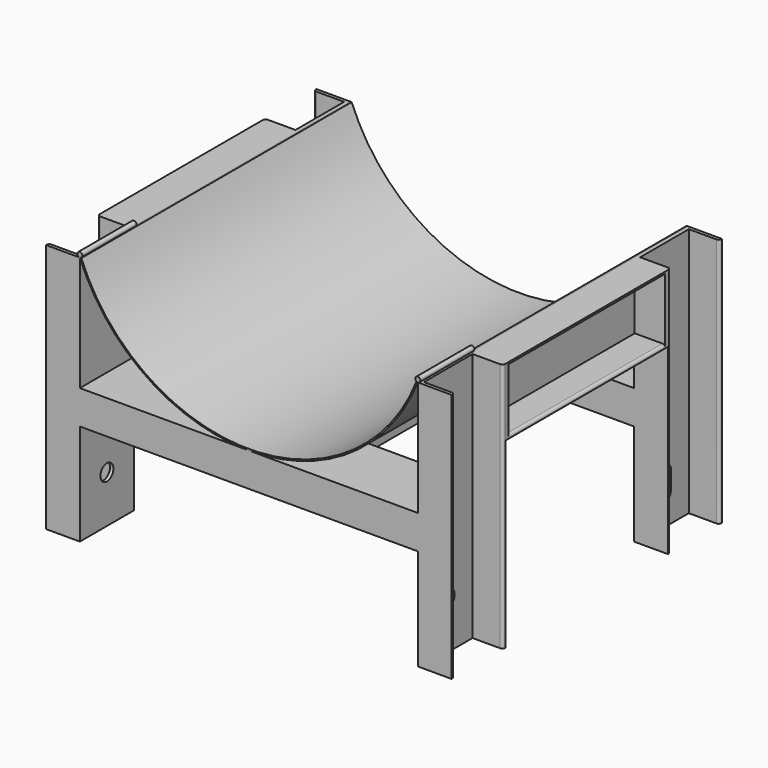
from build123d import *

# Parameters (mm, degrees)
F0_W      = 100
F0_H      = 150
F1_DEPTH  = 50
F2_T      = -5
F3_DEPTH  = 170
F4_DEPTH  = 200
F7_DEPTH  = 250
F8_W      = 300
F8_H      = 100
F9_DEPTH  = 50
F10_T     = -5
F11_R     = 4
F14_DEPTH = 555.001
F15_D     = 24
F16_R     = 3.75
F17_DEPTH = 100


# Not quite as in the source:
# - a feature names something its author has since deleted; it is built from what else it names


with BuildPart() as f1:
    # F0 (on Top) → F1 (new body)
    with BuildSketch(Plane.XY):
        Polygon((250, 250), (-250, 250), (-250, 150), (-50, 150), (50, 150), (250, 150), align=None)
        with Locations((0, 75)):
            Rectangle(F0_W, F0_H)
        with Locations((0, -75)):
            Rectangle(F0_W, F0_H)
        Polygon((50, -150), (-50, -150), (-250, -150), (-250, -250), (250, -250), (250, -150), align=None)
    extrude(amount=-F1_DEPTH)

    # F2
    f2_openings = [f1.faces().sort_by_distance(p)[0] for p in [
        (0, 0, -50),
    ]]
    offset(amount=F2_T, openings=f2_openings, kind=Kind.INTERSECTION)


with BuildPart() as f3:
    # F0 (on Top) → F3 (new body)
    with BuildSketch(Plane.XY):
        with BuildLine():
            Line((-250, -250), (-250, -150))
            Line((-250, -150), (-300, -150))
            Line((-300, -150), (-300, -151))
            ThreePointArc((-300, -151), (-298.8284271247, -153.8284271247), (-296, -155))
            Line((-296, -155), (-255, -155))
            Line((-255, -155), (-255, -245))
            Line((-255, -245), (-296, -245))
            ThreePointArc((-296, -245), (-298.8284271247, -246.1715728753), (-300, -249))
            Line((-300, -249), (-300, -250))
            Line((-300, -250), (-250, -250))
        make_face()
    extrude(amount=F3_DEPTH)


with BuildPart() as f3b:
    # F0 (on Top) → F3, piece 2 (new body)
    with BuildSketch(Plane.XY):
        with BuildLine():
            Line((300, -150), (250, -150))
            Line((250, -150), (250, -250))
            Line((250, -250), (300, -250))
            Line((300, -250), (300, -249))
            ThreePointArc((300, -249), (298.8284271247, -246.1715728753), (296, -245))
            Line((296, -245), (255, -245))
            Line((255, -245), (255, -155))
            Line((255, -155), (296, -155))
            ThreePointArc((296, -155), (298.8284271247, -153.8284271247), (300, -151))
            Line((300, -151), (300, -150))
        make_face()
    extrude(amount=F3_DEPTH)


with BuildPart() as f3c:
    # F0 (on Top) → F3, piece 3 (new body)
    with BuildSketch(Plane.XY):
        with BuildLine():
            Line((300, 250), (250, 250))
            Line((250, 250), (250, 150))
            Line((250, 150), (300, 150))
            Line((300, 150), (300, 151))
            ThreePointArc((300, 151), (298.8284271247, 153.8284271247), (296, 155))
            Line((296, 155), (255, 155))
            Line((255, 155), (255, 245))
            Line((255, 245), (296, 245))
            ThreePointArc((296, 245), (298.8284271247, 246.1715728753), (300, 249))
            Line((300, 249), (300, 250))
        make_face()
    extrude(amount=F3_DEPTH)


with BuildPart() as f3d:
    # F0 (on Top) → F3, piece 4 (new body)
    with BuildSketch(Plane.XY):
        with BuildLine():
            Line((-250, 150), (-250, 250))
            Line((-250, 250), (-300, 250))
            Line((-300, 250), (-300, 249))
            ThreePointArc((-300, 249), (-298.8284271247, 246.1715728753), (-296, 245))
            Line((-296, 245), (-255, 245))
            Line((-255, 245), (-255, 155))
            Line((-255, 155), (-296, 155))
            ThreePointArc((-296, 155), (-298.8284271247, 153.8284271247), (-300, 151))
            Line((-300, 151), (-300, 150))
            Line((-300, 150), (-250, 150))
        make_face()
    extrude(amount=F3_DEPTH)


with BuildPart() as f4:
    # F0 (on Top) → F4 (new body)
    with BuildSketch(Plane.XY):
        with BuildLine():
            Line((-250, -250), (-250, -150))
            Line((-250, -150), (-300, -150))
            Line((-300, -150), (-300, -151))
            ThreePointArc((-300, -151), (-298.8284271247, -153.8284271247), (-296, -155))
            Line((-296, -155), (-255, -155))
            Line((-255, -155), (-255, -245))
            Line((-255, -245), (-296, -245))
            ThreePointArc((-296, -245), (-298.8284271247, -246.1715728753), (-300, -249))
            Line((-300, -249), (-300, -250))
            Line((-300, -250), (-250, -250))
        make_face()
    extrude(amount=-F4_DEPTH)


with BuildPart() as f4b:
    # F0 (on Top) → F4, piece 2 (new body)
    with BuildSketch(Plane.XY):
        with BuildLine():
            Line((300, -150), (250, -150))
            Line((250, -150), (250, -250))
            Line((250, -250), (300, -250))
            Line((300, -250), (300, -249))
            ThreePointArc((300, -249), (298.8284271247, -246.1715728753), (296, -245))
            Line((296, -245), (255, -245))
            Line((255, -245), (255, -155))
            Line((255, -155), (296, -155))
            ThreePointArc((296, -155), (298.8284271247, -153.8284271247), (300, -151))
            Line((300, -151), (300, -150))
        make_face()
    extrude(amount=-F4_DEPTH)


with BuildPart() as f4c:
    # F0 (on Top) → F4, piece 3 (new body)
    with BuildSketch(Plane.XY):
        with BuildLine():
            Line((300, 250), (250, 250))
            Line((250, 250), (250, 150))
            Line((250, 150), (300, 150))
            Line((300, 150), (300, 151))
            ThreePointArc((300, 151), (298.8284271247, 153.8284271247), (296, 155))
            Line((296, 155), (255, 155))
            Line((255, 155), (255, 245))
            Line((255, 245), (296, 245))
            ThreePointArc((296, 245), (298.8284271247, 246.1715728753), (300, 249))
            Line((300, 249), (300, 250))
        make_face()
    extrude(amount=-F4_DEPTH)


with BuildPart() as f4d:
    # F0 (on Top) → F4, piece 4 (new body)
    with BuildSketch(Plane.XY):
        with BuildLine():
            Line((-250, 150), (-250, 250))
            Line((-250, 250), (-300, 250))
            Line((-300, 250), (-300, 249))
            ThreePointArc((-300, 249), (-298.8284271247, 246.1715728753), (-296, 245))
            Line((-296, 245), (-255, 245))
            Line((-255, 245), (-255, 155))
            Line((-255, 155), (-296, 155))
            ThreePointArc((-296, 155), (-298.8284271247, 153.8284271247), (-300, 151))
            Line((-300, 151), (-300, 150))
            Line((-300, 150), (-250, 150))
        make_face()
    extrude(amount=-F4_DEPTH)


with BuildPart() as f3b_1:
    add(f3b.part)

    # F5: union F4b, F3c, F4c, F3, F4, F4d, F3d, F1
    add(f4b.part)
    add(f3c.part)
    add(f4c.part)
    add(f3.part)
    add(f4.part)
    add(f4d.part)
    add(f3d.part)
    add(f1.part)



with BuildPart() as f7:
    # F6 (on Front) → F7 (new body, symmetric)
    with BuildSketch(Plane.XZ):
        with BuildLine():
            Line((-247.8481508552, 170), (-250, 170))
            ThreePointArc((-250, 170), (0, 0), (250, 170))
            Line((250, 170), (247.8481508552, 170))
            ThreePointArc((247.8481508552, 170), (0, 2), (-247.8481508552, 170))
        make_face()
    extrude(amount=F7_DEPTH, both=True)


with BuildPart() as f9:
    # F8 (on face) → F9 (new body)
    with BuildSketch(Plane(origin=(250, 0, 0), x_dir=(0, -1, 0), z_dir=(-1, 0, 0))):
        with Locations((0, 120)):
            Rectangle(F8_W, F8_H)
    extrude(amount=-F9_DEPTH)

    # F10
    f10_openings = [f9.faces().sort_by_distance(p)[0] for p in [
        (300, 0, 120),
    ]]
    offset(amount=F10_T, openings=f10_openings)

    # F11
    f11_edges = [f9.edges().sort_by_distance(p)[0] for p in [
        (300, 0, 165),
        (300, 0, 75),
    ]]
    fillet(f11_edges, radius=F11_R)


with BuildPart() as f3b_2:
    add(f3b_1.part)

    add(f9.part)  # F12 merges F9
    # F12: F9 across plane
    add(f9.part.mirror(Plane.YZ))

    # F13 (on face) → F14 (cut, through all)
    with BuildSketch(Plane.YZ.offset(255)):
        with BuildLine():
            ThreePointArc((212, -130), (208.4852813742, -121.5147186258), (200, -118))
            ThreePointArc((200, -118), (191.5147186258, -121.5147186258), (188, -130))
            Line((188, -130), (188, -156))
            ThreePointArc((188, -156), (191.5147186258, -164.4852813742), (200, -168))
            ThreePointArc((200, -168), (208.4852813742, -164.4852813742), (212, -156))
            Line((212, -156), (212, -130))
        make_face()
    extrude(amount=-F14_DEPTH, mode=Mode.SUBTRACT)

    # F15 (through all)
    with Locations(Plane.YZ.offset(255)):
        with Locations((-200, -130)):
            Hole(F15_D / 2)


with BuildPart() as f17:
    # F16 (on face) → F17 (new body)
    with BuildSketch(Plane.XZ.offset(250)):
        with Locations((-250, 173.75)):
            Circle(F16_R)
    extrude(amount=-F17_DEPTH)


with BuildPart() as f17b:
    # F16 (on face) → F17, piece 2 (new body)
    with BuildSketch(Plane.XZ.offset(250)):
        with Locations((250, 173.75)):
            Circle(F16_R)
    extrude(amount=-F17_DEPTH)


solid = Compound([f7.part, f3b_2.part, f17.part, f17b.part])
